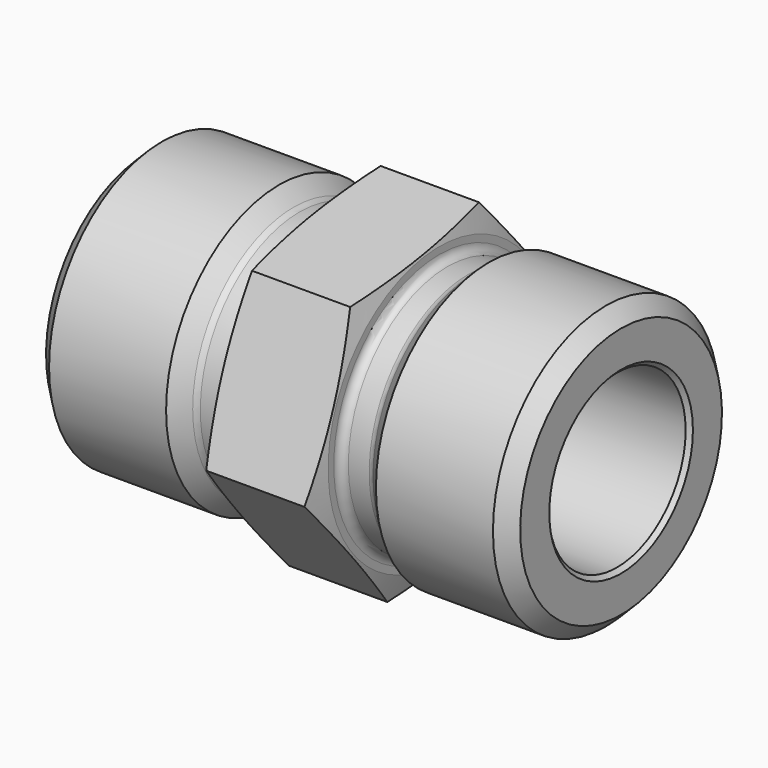
from build123d import *

# Parameters (mm, degrees)
F2_SIZE2       = 0.75
F2_SIZE        = 0.75
F3_R           = 0.4
F7_DEPTH       = 2.75
F7_DEPTH_BACK  = 2.75
F8_R           = 0.4
F13_R          = 4.25
F14_DEPTH      = 25
F14_DEPTH_BACK = 44
F15_SIZE2      = 0.2
F15_SIZE       = 0.2


# Not quite as in the source:
# - an extrude ends at something that could not be found from the text; its depth is read off the source's solid


with BuildPart() as f1:
    # F0 (on Front) → F1 (revolve)
    with BuildSketch(Plane.XZ):
        Polygon((0, 6.15), (0, 0), (11.75, 0), (11.75, 7), (5.2, 7), (4.35, 6.15), (2.75, 6.15), align=None)
    revolve(axis=Axis((5.875, 0, 0), (-1, 0, 0)))

    # F2
    f2_edges = [f1.edges().sort_by_distance(p)[0] for p in [
        (11.75, 0, -7),
    ]]
    chamfer(f2_edges, length=F2_SIZE, length2=F2_SIZE2)

    # F3
    f3_edges = [f1.edges().sort_by_distance(p)[0] for p in [
        (4.35, 0, -6.15),
    ]]
    fillet(f3_edges, radius=F3_R)

    # F4: F1 across plane


with BuildPart() as f1_1:
    add(f1.part)
    add(f1.part.mirror(Plane.XZ))

    # F5: F1 across plane


with BuildPart() as f1_2:
    add(f1_1.part)
    add(f1_1.part.mirror(Plane.YZ))

    # F6 (on Right) → F7 (join, two sides)
    with BuildSketch(Plane.YZ) as f7_sk:
        Polygon((2.834367898, 7.5696559996), (-5.1383304446, 6.2394626031), (-7.9726983425, -1.3301933965), (-2.834367898, -7.5696559996), (5.1383304446, -6.2394626031), (7.9726983425, 1.3301933965), align=None)
    extrude(amount=F7_DEPTH)
    extrude(f7_sk.sketch, amount=-F7_DEPTH_BACK)

    # F8
    f8_edges = [f1_2.edges().sort_by_distance(p)[0] for p in [
        (-2.75, 0, -6.15),
        (2.75, 0, -6.15),
    ]]
    fillet(f8_edges, radius=F8_R)


with BuildPart() as f10:
    # F9 (on Top) → F10 (revolve)
    with BuildSketch(Plane.XY):
        Polygon((-5.5153914727, 9.7084684995), (-2.75, 6.9), (-1.9974731336, 9.7084684995), align=None)
    revolve(axis=Axis((-5.9099821374, 0, 0), (1, 0, 0)))


with BuildPart() as f11_1:
    # F11: instance of F10
    add(f10.part.mirror(Plane.YZ))


with BuildPart() as f1_3:
    add(f1_2.part)

    # F12: cut F10, F11_1
    add(f10.part, mode=Mode.SUBTRACT)
    add(f11_1.part, mode=Mode.SUBTRACT)

    # F13 (on face) → F14 (cut, two sides)
    with BuildSketch(Plane.YZ.offset(11.75)) as f14_sk:
        Circle(F13_R)
    extrude(amount=-F14_DEPTH, mode=Mode.SUBTRACT)
    extrude(f14_sk.sketch, amount=F14_DEPTH_BACK, mode=Mode.SUBTRACT)

    # F15
    f15_edges = [f1_3.edges().sort_by_distance(p)[0] for p in [
        (11.75, -4.25, 0),
        (-11.75, -4.25, 0),
    ]]
    chamfer(f15_edges, length=F15_SIZE, length2=F15_SIZE2)


solid = f1_3.part
